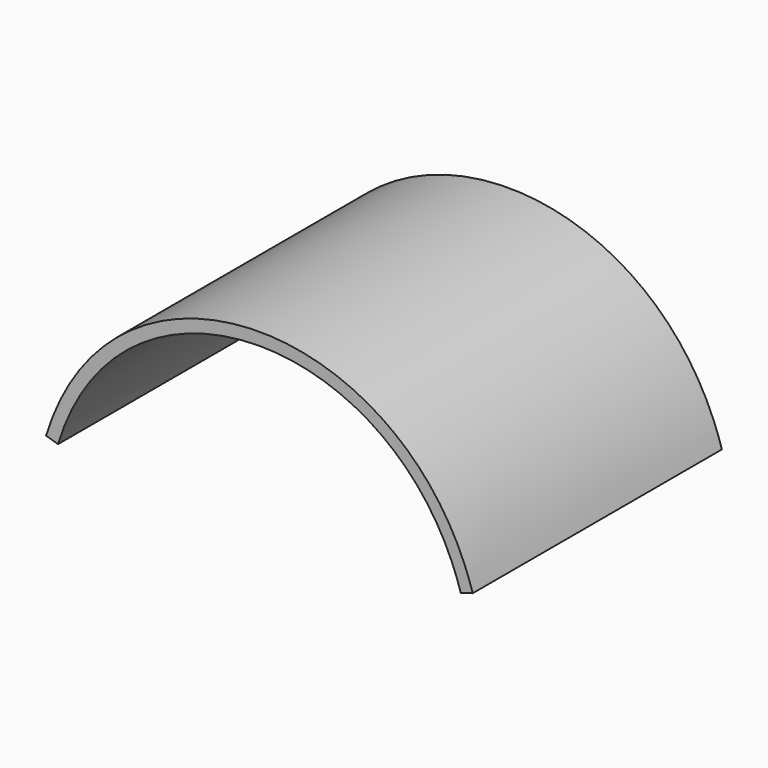
from build123d import *

# Parameters (mm, degrees)
F1_DEPTH = 25


with BuildPart() as f1:
    # F0 (on Front) → F1 (new body)
    with BuildSketch(Plane.XZ):
        with BuildLine():
            Line((-17.1202543454, 0.2929149433), (-16.1641158429, 0))
            add(Edge.make_bspline(
                [(-16.1641158429, 0), (-11.1782272682, 16.2750318656), (11.1782272682, 16.2750318656), (16.1641158429, 0)],
                knots=[0, 0, 0, 0, 32.3282316857, 32.3282316857, 32.3282316857, 32.3282316857], degree=3))
            Line((16.1641158429, 0), (17.1202543454, 0.2929149433))
            add(Edge.make_bspline(
                [(-17.1202543454, 0.2929149433), (-16.4663645681, 2.4273543319), (-14.5791189005, 6.1895876945), (-10.4313726901, 10.241968629), (-5.4244559822, 12.6685663001), (0, 13.4751276988), (5.4244559822, 12.6685663001), (10.4313726901, 10.241968629), (14.5791189005, 6.1895876945), (16.4663645681, 2.4273543319), (17.1202543454, 0.2929149433)],
                knots=[0, 0, 0, 0, 0.125, 0.25, 0.375, 0.5, 0.625, 0.75, 0.875, 1, 1, 1, 1], degree=3))
        make_face()
    extrude(amount=F1_DEPTH)


solid = f1.part
